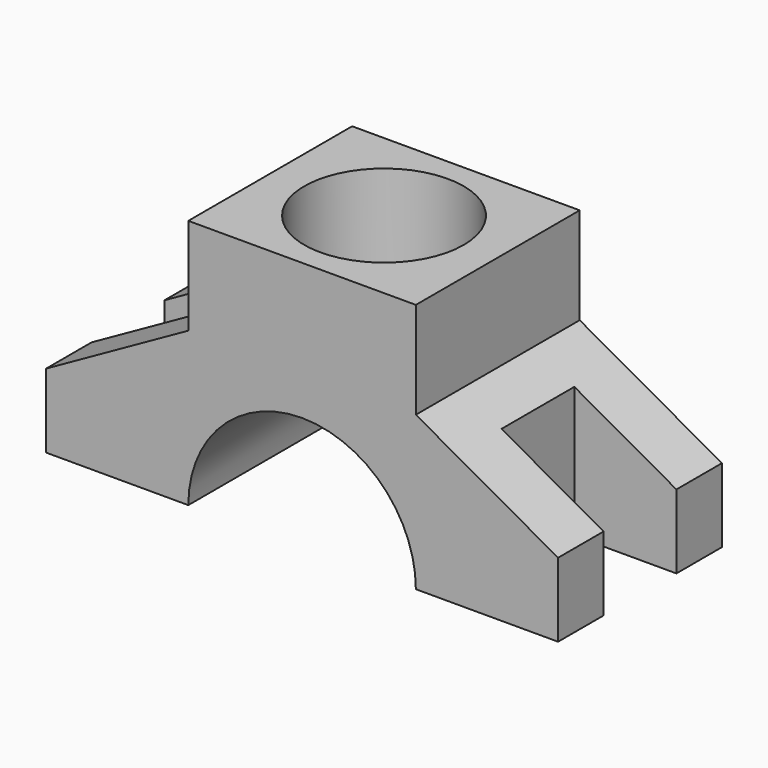
from build123d import *

# Parameters (mm, degrees)
F1_DEPTH = 36
F3_DEPTH = 36
F4_R     = 14
F4_W     = 18
F4_H     = 16
F5_DEPTH = 44


with BuildPart() as f1:
    # F0 (on Front) → F1 (new body)
    with BuildSketch(Plane.XZ):
        Polygon((0, 44), (0, 0), (45, 0), (45, 13), (20, 27), (20, 44), align=None)
        Polygon((-45, 0), (0, 0), (0, 44), (-20, 44), (-20, 27), (-45, 13), align=None)
    extrude(amount=-F1_DEPTH)

    # F2 (on face) → F3 (cut)
    with BuildSketch(Plane.XZ):
        with BuildLine():
            Line((-20, 0), (20, 0))
            ThreePointArc((20, 0), (0, 20), (-20, 0))
        make_face()
    extrude(amount=-F3_DEPTH, mode=Mode.SUBTRACT)

    # F4 (on Top) → F5 (cut)
    with BuildSketch(Plane.XY):
        with Locations((0, 18)):
            Circle(F4_R)
        with Locations((-36.059196651, 18)):
            Rectangle(F4_W, F4_H)
        with Locations((36.059196651, 18)):
            Rectangle(F4_W, F4_H)
    extrude(amount=F5_DEPTH, mode=Mode.SUBTRACT)


solid = f1.part
